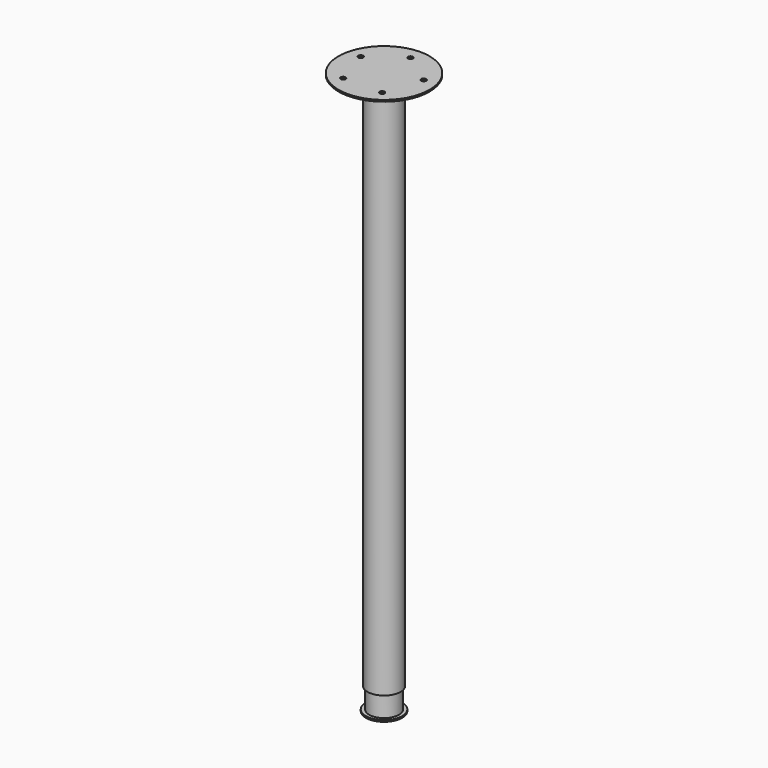
from build123d import *

# Parameters (mm, degrees)
F0_R            = 55
F1_DEPTH        = 2
F2_R            = 20
F2_R_2          = 18
F3_DEPTH        = 650
F4_R            = 18
F4_R_2          = 16
F5_DEPTH        = 25
F5_DEPTH_BACK   = 25
F6_R            = 22
F7_DEPTH        = 2
F8_R            = 3
F9_DEPTH        = 2.001
F9_COPIES_COUNT = 5


# Not quite as in the source:
# - a pattern or mirror of a feature is missing from the dataset's text; its kind, count and spacing are read off the source's solid


with BuildPart() as f1:
    # F0 (on Top) → F1 (new body)
    with BuildSketch(Plane.XY):
        Circle(F0_R)
    extrude(amount=F1_DEPTH)

    # F2 (on face) → F3 (join)
    with BuildSketch(Plane(origin=(0, 0, 0), x_dir=(1, 0, 0), z_dir=(0, 0, -1))):
        Circle(F2_R)
        Circle(F2_R_2, mode=Mode.SUBTRACT)
    extrude(amount=F3_DEPTH)

    # F4 (on face) → F5 (join, two sides)
    with BuildSketch(Plane(origin=(0, 0, -650), x_dir=(1, 0, 0), z_dir=(0, 0, -1))) as f5_sk:
        Circle(F4_R)
        Circle(F4_R_2, mode=Mode.SUBTRACT)
    extrude(amount=F5_DEPTH)
    extrude(f5_sk.sketch, amount=-F5_DEPTH_BACK)

    # F6 (on face) → F7 (join)
    with BuildSketch(Plane(origin=(0, 0, -675), x_dir=(1, 0, 0), z_dir=(0, 0, -1))):
        Circle(F6_R)
    extrude(amount=F7_DEPTH)

    # F8 (on face) → F9 (cut, through all)
    with BuildSketch(Plane(origin=(0, 0, 0), x_dir=(1, 0, 0), z_dir=(0, 0, -1))):
        with Locations((0, -40)):
            Circle(F8_R)
    f9 = extrude(amount=-F9_DEPTH, mode=Mode.SUBTRACT)

    # F9_copies: F9 ×5 about axis
    f9_copies_axis = Axis((0, 0, 0), (0, 0, 1))
    for i in range(1, F9_COPIES_COUNT):
        add(f9.rotate(f9_copies_axis, i * 360 / F9_COPIES_COUNT), mode=Mode.SUBTRACT)


solid = f1.part
